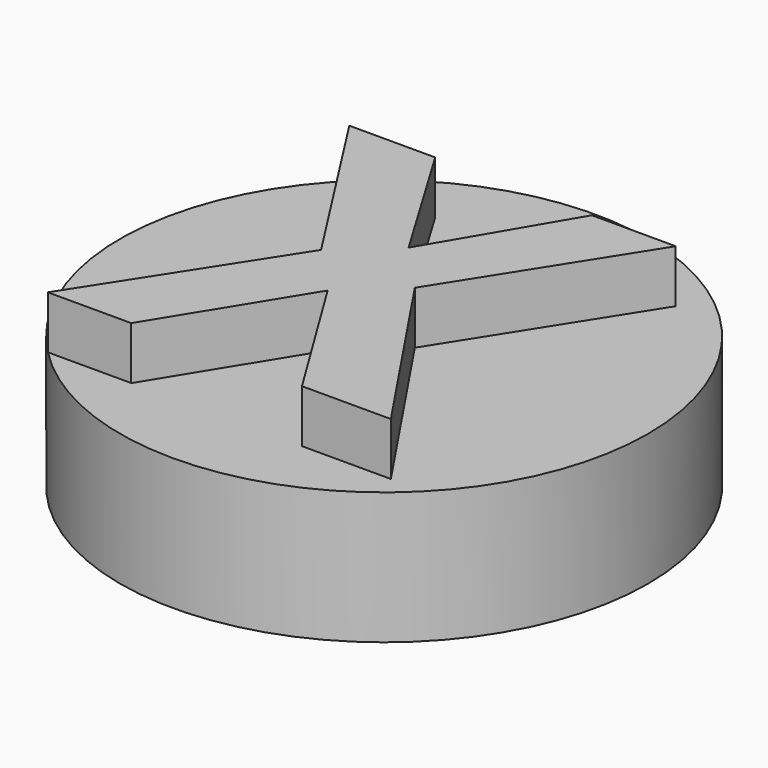
from build123d import *

# Parameters (mm, degrees)
F0_R         = 12.7
F1_DEPTH     = 6.35
F2_TEXT_SIZE = 24.7402999805
F3_DEPTH     = 2.54


# Not quite as in the source:
# - Text() gives the source's letters only with a copy of the font that has no kerning and outlines rounded to 1/6400 em; it was checked with that copy


with BuildPart() as f1:
    # F0 (on Top) → F1 (new body)
    with BuildSketch(Plane.XY):
        Circle(F0_R)
    extrude(amount=F1_DEPTH)

    # F2 (on face) → F3 (join)
    with BuildSketch(Plane.XY.offset(6.35)):
        with Locations((-9.0534035241, -8.906507993)):
            Text('X', F2_TEXT_SIZE, font='Open Sans', font_style=FontStyle.BOLD, text_align=(TextAlign.LEFT, TextAlign.BOTTOM))
    extrude(amount=F3_DEPTH)


solid = f1.part
